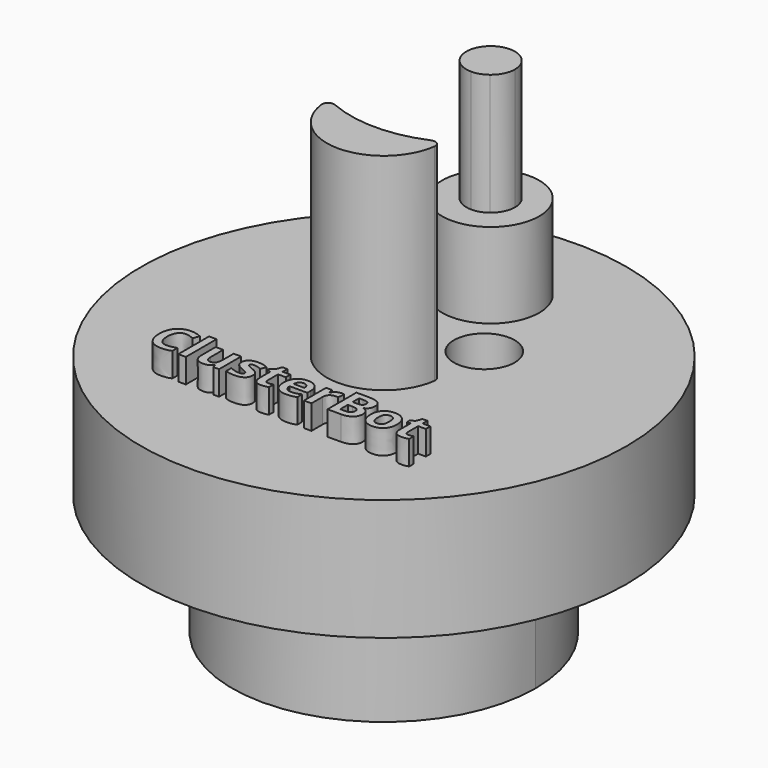
from build123d import *

# Parameters (mm, degrees)
F0_R          = 20
F1_DEPTH      = 10
F2_DEPTH      = 27
F3_DEPTH      = 10
F3_DEPTH_BACK = 10
F4_DEPTH      = 10
F5_R          = 0.5
F6_R          = 1.55
F7_DEPTH      = 10
F6_R_2        = 2.5
F8_DEPTH      = 6
F9_TEXT_SIZE  = 4.1666666667
F10_DEPTH     = 2
F11_R         = 4
F12_DEPTH     = 7
F13_DEPTH     = 3


# Not quite as in the source:
# - a feature names something its author has since deleted; it is built from what else it names
# - Text() gives the source's letters only with a copy of the font that has no kerning and outlines rounded to 1/6400 em; it was checked with that copy


with BuildPart() as f1:
    # F0 (on Top) → F1 (new body)
    with BuildSketch(Plane.XY):
        Circle(F0_R)
        with BuildLine():
            ThreePointArc((-1.4079449152, 12.4204545455), (0, 13), (1.4079449152, 12.4204545455))
            ThreePointArc((1.4079449152, 12.4204545455), (9.3233393009, 8.3261842569), (12.5, 0))
            ThreePointArc((12.5, 0), (-8.3261842569, -9.3233393009), (-1.4079449152, 12.4204545455))
        make_face(mode=Mode.SUBTRACT)
    extrude(amount=F1_DEPTH)



with BuildPart() as f1b:
    # F0 (on Top) → F1, piece 2 (new body)
    with BuildSketch(Plane.XY):
        with BuildLine():
            ThreePointArc((9.5, 0), (7.1380876968, 6.2687880832), (1.2267991511, 9.4204545455))
            ThreePointArc((1.2267991511, 9.4204545455), (0.6484246644, 9.1080313283), (0, 9))
            ThreePointArc((0, 9), (-0.6484246644, 9.1080313283), (-1.2267991511, 9.4204545455))
            ThreePointArc((-1.2267991511, 9.4204545455), (-6.2687880832, -7.1380876968), (9.5, 0))
        make_face()
        with BuildLine():
            ThreePointArc((-4.6924006055, 0.2671639152), (-3.2275632913, 3.4165531169), (0, 4.7))
            ThreePointArc((0, 4.7), (3.2275632913, 3.4165531169), (4.6924006055, 0.2671639152))
            ThreePointArc((4.6924006055, 0.2671639152), (4.6980997672, 0.1336359873), (4.7, 0))
            ThreePointArc((4.7, 0), (-0.1336359873, -4.6980997672), (-4.6924006055, 0.2671639152))
        make_face(mode=Mode.SUBTRACT)
        with BuildLine():
            ThreePointArc((4.6924006055, 0.2671639152), (3.2275632913, 3.4165531169), (0, 4.7))
            ThreePointArc((0, 4.7), (-3.2275632913, 3.4165531169), (-4.6924006055, 0.2671639152))
            ThreePointArc((-4.6924006055, 0.2671639152), (0, -0.9021296262), (4.6924006055, 0.2671639152))
        make_face()
        with BuildLine():
            ThreePointArc((4.7, 0), (4.6980997672, 0.1336359873), (4.6924006055, 0.2671639152))
            ThreePointArc((4.6924006055, 0.2671639152), (0, -0.9021296262), (-4.6924006055, 0.2671639152))
            ThreePointArc((-4.6924006055, 0.2671639152), (-0.1336359873, -4.6980997672), (4.7, 0))
        make_face()
    extrude(amount=F1_DEPTH)


with BuildPart() as f1_1:
    add(f1.part)

    add(f1b.part)  # F2 merges F1b
    # F0 (on Top) → F2 (join)
    with BuildSketch(Plane.XY):
        with BuildLine():
            ThreePointArc((1.2267991511, 9.4204545455), (1.7963293548, 10.1206815998), (2, 11))
            ThreePointArc((2, 11), (1.846062002, 11.7694511582), (1.4079449152, 12.4204545455))
            ThreePointArc((1.4079449152, 12.4204545455), (0, 12.5), (-1.4079449152, 12.4204545455))
            ThreePointArc((-1.4079449152, 12.4204545455), (-1.9963639632, 10.8794557081), (-1.2267991511, 9.4204545455))
            ThreePointArc((-1.2267991511, 9.4204545455), (-0.6146876516, 9.4800927786), (0, 9.5))
            ThreePointArc((0, 9.5), (0.6146876516, 9.4800927786), (1.2267991511, 9.4204545455))
        make_face()
        with BuildLine():
            ThreePointArc((-1.4079449152, 12.4204545455), (0, 12.5), (1.4079449152, 12.4204545455))
            ThreePointArc((1.4079449152, 12.4204545455), (0, 13), (-1.4079449152, 12.4204545455))
        make_face()
        with BuildLine():
            ThreePointArc((0, 9), (0.6484246644, 9.1080313283), (1.2267991511, 9.4204545455))
            ThreePointArc((1.2267991511, 9.4204545455), (0.6146876516, 9.4800927786), (0, 9.5))
            Line((0, 9.5), (0, 9))
        make_face()
        with BuildLine():
            ThreePointArc((-1.2267991511, 9.4204545455), (-0.6484246644, 9.1080313283), (0, 9))
            Line((0, 9), (0, 9.5))
            ThreePointArc((0, 9.5), (-0.6146876516, 9.4800927786), (-1.2267991511, 9.4204545455))
        make_face()
        with BuildLine():
            ThreePointArc((4.7, 0), (4.6980997672, 0.1336359873), (4.6924006055, 0.2671639152))
            ThreePointArc((4.6924006055, 0.2671639152), (0, -0.9021296262), (-4.6924006055, 0.2671639152))
            ThreePointArc((-4.6924006055, 0.2671639152), (-0.1336359873, -4.6980997672), (4.7, 0))
        make_face()
    extrude(amount=F2_DEPTH)

    # F0 (on Top) → F3 (join, two sides)
    with BuildSketch(Plane.XY) as f3_sk:
        with BuildLine():
            ThreePointArc((1.4079449152, 12.4204545455), (1.846062002, 11.7694511582), (2, 11))
            ThreePointArc((2, 11), (1.7963293548, 10.1206815998), (1.2267991511, 9.4204545455))
            ThreePointArc((1.2267991511, 9.4204545455), (7.1380876968, 6.2687880832), (9.5, 0))
            ThreePointArc((9.5, 0), (-6.2687880832, -7.1380876968), (-1.2267991511, 9.4204545455))
            ThreePointArc((-1.2267991511, 9.4204545455), (-1.9963639632, 10.8794557081), (-1.4079449152, 12.4204545455))
            ThreePointArc((-1.4079449152, 12.4204545455), (-8.3261842569, -9.3233393009), (12.5, 0))
            ThreePointArc((12.5, 0), (9.3233393009, 8.3261842569), (1.4079449152, 12.4204545455))
        make_face()
    extrude(amount=-F3_DEPTH)
    extrude(f3_sk.sketch, amount=F3_DEPTH_BACK)

    # F0 (on Top) → F4 (join)
    with BuildSketch(Plane.XY):
        with BuildLine():
            ThreePointArc((1.2267991511, 9.4204545455), (1.7963293548, 10.1206815998), (2, 11))
            ThreePointArc((2, 11), (1.846062002, 11.7694511582), (1.4079449152, 12.4204545455))
            ThreePointArc((1.4079449152, 12.4204545455), (0, 12.5), (-1.4079449152, 12.4204545455))
            ThreePointArc((-1.4079449152, 12.4204545455), (-1.9963639632, 10.8794557081), (-1.2267991511, 9.4204545455))
            ThreePointArc((-1.2267991511, 9.4204545455), (-0.6146876516, 9.4800927786), (0, 9.5))
            ThreePointArc((0, 9.5), (0.6146876516, 9.4800927786), (1.2267991511, 9.4204545455))
        make_face()
    extrude(amount=-F4_DEPTH)

    # F5
    f5_edges = [f1_1.edges().sort_by_distance(p)[0] for p in [
        (-4.692401, 0.267164, 18.5),
        (4.692401, 0.267164, 18.5),
    ]]
    fillet(f5_edges, radius=F5_R)

    # F6 (on face) → F7 (cut)
    with BuildSketch(Plane.XY.offset(10)):
        with Locations((-4.5961940777, 4.5961940777)):
            Circle(F6_R)
        with Locations((4.5961940777, 4.5961940777)):
            Circle(F6_R)
    extrude(amount=-F7_DEPTH, mode=Mode.SUBTRACT)

    # F6 (on face) → F8 (cut)
    with BuildSketch(Plane.XY.offset(10)):
        with Locations((4.5961940777, 4.5961940777)):
            Circle(F6_R_2)
        with Locations((4.5961940777, 4.5961940777)):
            Circle(F6_R, mode=Mode.SUBTRACT)
        with Locations((-4.5961940777, 4.5961940777)):
            Circle(F6_R_2)
        with Locations((-4.5961940777, 4.5961940777)):
            Circle(F6_R, mode=Mode.SUBTRACT)
    extrude(amount=-F8_DEPTH, mode=Mode.SUBTRACT)

    # F9 (on face) → F10 (join)
    with BuildSketch(Plane.XY.offset(10)):
        with Locations((-11.1110026042, -11)):
            Text('ClusterBot', F9_TEXT_SIZE, font='Open Sans', font_style=FontStyle.BOLD, text_align=(TextAlign.LEFT, TextAlign.BOTTOM))
    extrude(amount=F10_DEPTH)

    # F11 (on face) → F12 (join)
    with BuildSketch(Plane.XY.offset(10)):
        with Locations((0, 11)):
            Circle(F11_R)
    extrude(amount=F12_DEPTH)

    # F13 (add): a face of the model
    f13_faces = [f1_1.faces().sort_by_distance(p)[0] for p in [
        (0, -0.2584669968, 0),
    ]]
    extrude(f13_faces, amount=F13_DEPTH)


solid = f1_1.part
